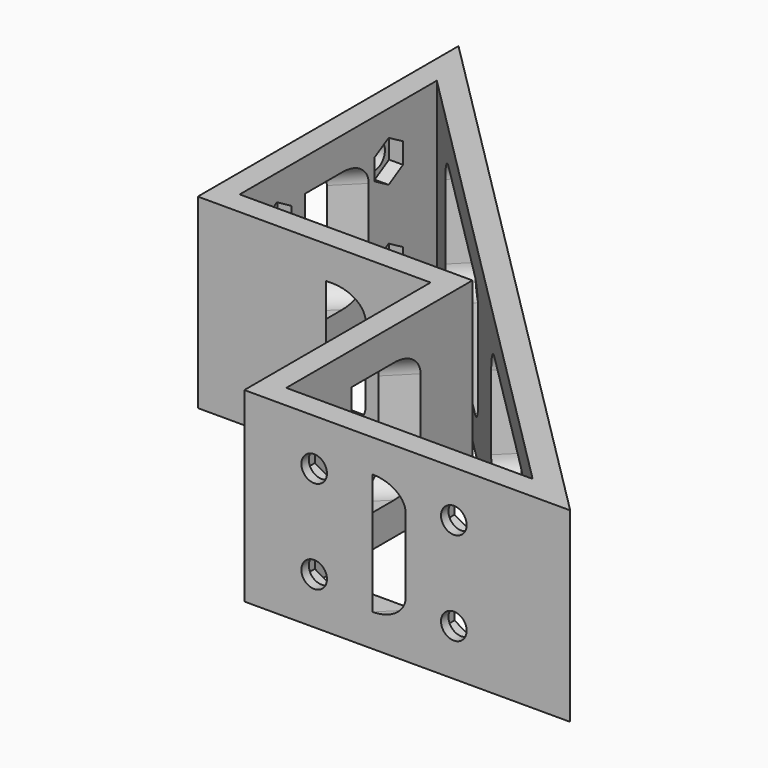
from build123d import *

# Parameters (mm, degrees)
F1_DEPTH  = 40
F2_T      = -5
F4_DEPTH  = 30
F5_R      = 2.75
F6_DEPTH  = 5
F7_R      = 2.75
F8_DEPTH  = 5
F9_R      = 2.75
F10_DEPTH = 3
F11_R     = 2.75
F12_DEPTH = 3


# Not quite as in the source:
# - a feature names something its author has since deleted; it is built from what else it names


with BuildPart() as f1:
    # F0 (on Top) → F1 (new body)
    with BuildSketch(Plane.XY):
        Polygon((120, 0), (0, 120), (0, 100), (50, 50), (100, 0), align=None)
        Polygon((50, 50), (0, 100), (0, 92.9289321881), (42.9289321881, 50), align=None)
        Polygon((42.9289321881, 50), (0, 92.9289321881), (0, 50), align=None)
        Polygon((92.9289321881, 0), (50, 42.9289321881), (50, 0), align=None)
        Polygon((100, 0), (50, 50), (50, 42.9289321881), (92.9289321881, 0), align=None)
    extrude(amount=F1_DEPTH)

    # F2
    f2_openings = [f1.faces().sort_by_distance(p)[0] for p in [
        (51.697056, 25, 40),
        (51.697056, 25, 0),
    ]]
    offset(amount=F2_T, openings=f2_openings, kind=Kind.INTERSECTION)

    # F3 (on face) → F4 (cut)
    with BuildSketch(Plane(origin=(60, 60, 0), x_dir=(-0.7071067812, 0.7071067812, 0), z_dir=(0.7071067812, 0.7071067812, 0))):
        with BuildLine():
            ThreePointArc((59.8528137424, 28), (58.3883476483, 31.5355339059), (54.8528137424, 33))
            Line((54.8528137424, 33), (14.8528137424, 33))
            ThreePointArc((14.8528137424, 33), (11.3172798365, 31.5355339059), (9.8528137424, 28))
            Line((9.8528137424, 28), (9.8528137424, 12))
            ThreePointArc((9.8528137424, 12), (11.3172798365, 8.4644660941), (14.8528137424, 7))
            Line((14.8528137424, 7), (54.8528137424, 7))
            ThreePointArc((54.8528137424, 7), (58.3883476483, 8.4644660941), (59.8528137424, 12))
            Line((59.8528137424, 12), (59.8528137424, 28))
        make_face()
        with BuildLine():
            ThreePointArc((-54.8528137424, 33), (-58.3883476483, 31.5355339059), (-59.8528137424, 28))
            Line((-59.8528137424, 28), (-59.8528137424, 12))
            ThreePointArc((-59.8528137424, 12), (-58.3883476483, 8.4644660941), (-54.8528137424, 7))
            Line((-54.8528137424, 7), (-14.8528137424, 7))
            ThreePointArc((-14.8528137424, 7), (-11.3172798365, 8.4644660941), (-9.8528137424, 12))
            Line((-9.8528137424, 12), (-9.8528137424, 28))
            ThreePointArc((-9.8528137424, 28), (-11.3172798365, 31.5355339059), (-14.8528137424, 33))
            Line((-14.8528137424, 33), (-54.8528137424, 33))
        make_face()
    extrude(amount=-F4_DEPTH, mode=Mode.SUBTRACT)

    # F5 (on face) → F6 (cut, through all)
    with BuildSketch(Plane(origin=(0, 0, 0), x_dir=(0, -1, 0), z_dir=(-1, 0, 0))):
        with Locations((-95, 10)):
            Circle(F5_R)
        with Locations((-95, 30)):
            Circle(F5_R)
        with Locations((-65, 10)):
            Circle(F5_R)
        with Locations((-65, 30)):
            Circle(F5_R)
    extrude(amount=-F6_DEPTH, mode=Mode.SUBTRACT)

    # F7 (on face) → F8 (cut, through all)
    with BuildSketch(Plane.XZ):
        with Locations((65, 30)):
            Circle(F7_R)
        with Locations((95, 30)):
            Circle(F7_R)
        with Locations((95, 10)):
            Circle(F7_R)
        with Locations((65, 10)):
            Circle(F7_R)
    extrude(amount=-F8_DEPTH, mode=Mode.SUBTRACT)

    # F9 (on face) → F10 (cut)
    with BuildSketch(Plane.YZ.offset(5)):
        Polygon((61.15, 27.7772014636), (65, 25.5544029272), (68.85, 27.7772014636), (68.85, 32.2227985364), (65, 34.4455970728), (61.15, 32.2227985364), align=None)
        with Locations((65, 30)):
            Circle(F9_R, mode=Mode.SUBTRACT)
        Polygon((61.15, 12.2227985364), (61.15, 7.7772014636), (65, 5.5544029272), (68.85, 7.7772014636), (68.85, 12.2227985364), (65, 14.4455970728), align=None)
        with Locations((65, 10)):
            Circle(F9_R, mode=Mode.SUBTRACT)
        Polygon((91.15, 7.7772014636), (95, 5.5544029272), (98.85, 7.7772014636), (98.85, 12.2227985364), (95, 14.4455970728), (91.15, 12.2227985364), align=None)
        with Locations((95, 10)):
            Circle(F9_R, mode=Mode.SUBTRACT)
        Polygon((91.15, 27.7772014636), (95, 25.5544029272), (98.85, 27.7772014636), (98.85, 32.2227985364), (95, 34.4455970728), (91.15, 32.2227985364), align=None)
        with Locations((95, 30)):
            Circle(F9_R, mode=Mode.SUBTRACT)
    extrude(amount=-F10_DEPTH, mode=Mode.SUBTRACT)

    # F11 (on face) → F12 (cut)
    with BuildSketch(Plane(origin=(0, 5, 0), x_dir=(-1, 0, 0), z_dir=(0, 1, 0))):
        Polygon((-91.15, 12.2227985364), (-95, 14.4455970728), (-98.85, 12.2227985364), (-98.85, 7.7772014636), (-95, 5.5544029272), (-91.15, 7.7772014636), align=None)
        with Locations((-95, 10)):
            Circle(F11_R, mode=Mode.SUBTRACT)
        Polygon((-91.15, 32.2227985364), (-95, 34.4455970728), (-98.85, 32.2227985364), (-98.85, 27.7772014636), (-95, 25.5544029272), (-91.15, 27.7772014636), align=None)
        with Locations((-95, 30)):
            Circle(F11_R, mode=Mode.SUBTRACT)
        Polygon((-61.15, 32.2227985364), (-65, 34.4455970728), (-68.85, 32.2227985364), (-68.85, 27.7772014636), (-65, 25.5544029272), (-61.15, 27.7772014636), align=None)
        with Locations((-65, 30)):
            Circle(F11_R, mode=Mode.SUBTRACT)
        Polygon((-61.15, 12.2227985364), (-65, 14.4455970728), (-68.85, 12.2227985364), (-68.85, 7.7772014636), (-65, 5.5544029272), (-61.15, 7.7772014636), align=None)
        with Locations((-65, 10)):
            Circle(F11_R, mode=Mode.SUBTRACT)
    extrude(amount=-F12_DEPTH, mode=Mode.SUBTRACT)


solid = f1.part
